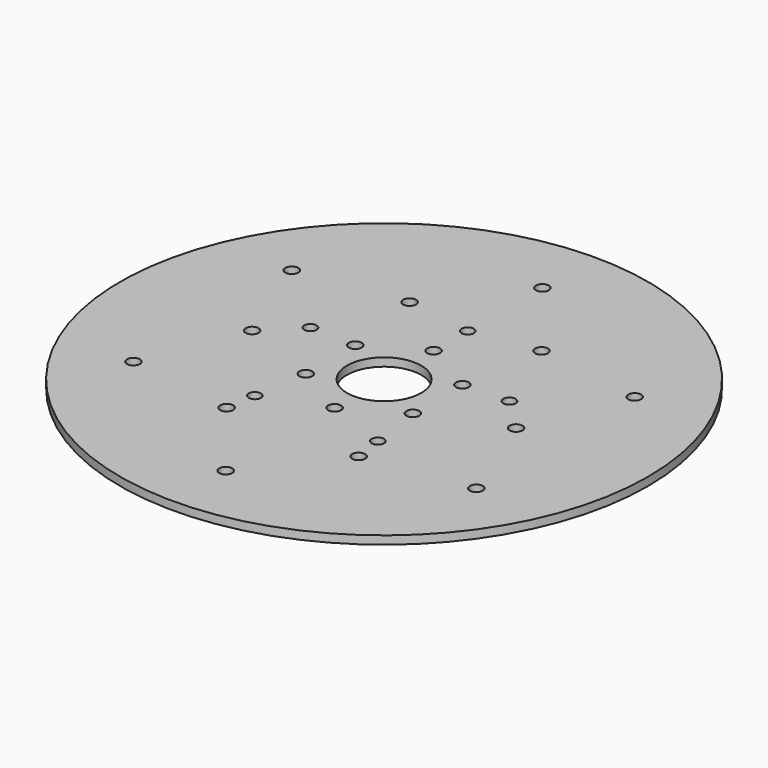
from build123d import *

# Parameters (mm, degrees)
F0_R            = 101.6
F0_R_2          = 14.2875
F1_DEPTH        = 3.175
F2_R            = 2.4892
F3_DEPTH        = 3.176
F3_COPIES_COUNT = 6
F4_R            = 2.3622
F5_DEPTH        = 3.176


# Not quite as in the source:
# - a pattern or mirror of a feature is missing from the dataset's text; its kind, count and spacing are read off the source's solid


with BuildPart() as f1:
    # F0 (on Top) → F1 (new body)
    with BuildSketch(Plane.XY):
        Circle(F0_R)
        Circle(F0_R_2, mode=Mode.SUBTRACT)
    extrude(amount=F1_DEPTH)

    # F2 (on face) → F3 (cut, through all)
    with BuildSketch(Plane.XY.offset(3.175)):
        with Locations((0, 23.8125)):
            Circle(F2_R)
        with Locations((0, 76.2)):
            Circle(F2_R)
        with Locations((25.4, 43.9940905122)):
            Circle(F2_R)
    f3 = extrude(amount=-F3_DEPTH, mode=Mode.SUBTRACT)

    # F3_copies: F3 ×6 about axis
    f3_copies_axis = Axis((0, 0, 0), (0, 0, 1))
    for i in range(1, F3_COPIES_COUNT):
        add(f3.rotate(f3_copies_axis, i * 360 / F3_COPIES_COUNT), mode=Mode.SUBTRACT)

    # F4 (on face) → F5 (cut, through all)
    with BuildSketch(Plane.XY.offset(3.175)):
        with Locations((0, 40.2743678674)):
            Circle(F4_R)
        with Locations((38.3032, 12.4454641087)):
            Circle(F4_R)
        with Locations((23.6726794779, -32.5826480425)):
            Circle(F4_R)
        with Locations((-23.6726794779, -32.5826480425)):
            Circle(F4_R)
        with Locations((-38.3032, 12.4454641087)):
            Circle(F4_R)
    extrude(amount=-F5_DEPTH, mode=Mode.SUBTRACT)


solid = f1.part
